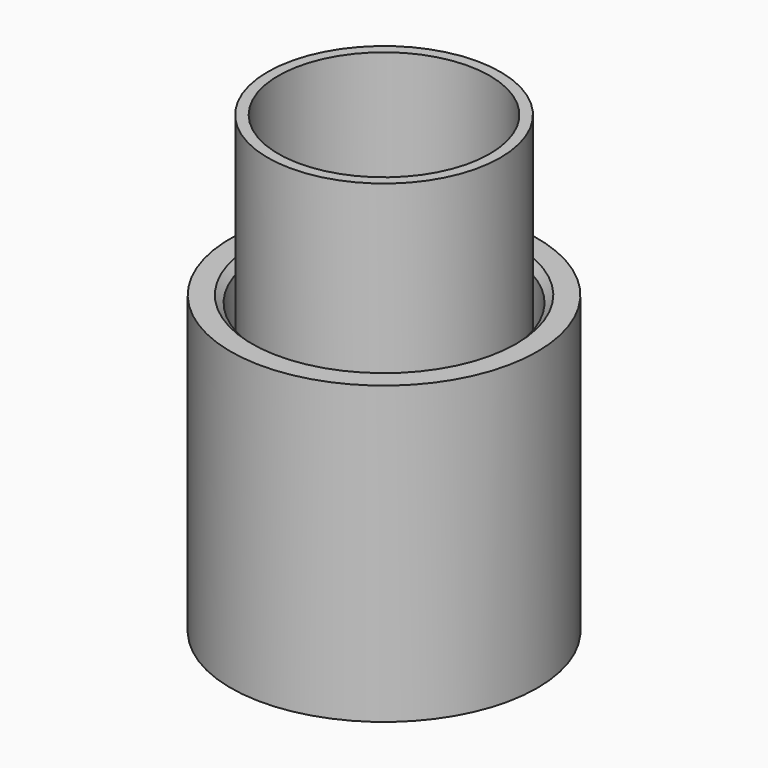
from build123d import *

# Parameters (mm, degrees)
F0_R     = 11
F0_R_2   = 10
F1_DEPTH = 40
F2_R     = 14.5
F2_R_2   = 11.5
F3_DEPTH = 25
F4_R     = 14.5
F5_DEPTH = 3
F6_SIZE  = 1
F7_SIZE2 = 5
F7_SIZE  = 0.5


with BuildPart() as f1:
    # F0 (on Top) → F1 (new body)
    with BuildSketch(Plane.XY):
        Circle(F0_R)
        Circle(F0_R_2, mode=Mode.SUBTRACT)
    extrude(amount=F1_DEPTH)


with BuildPart() as f3:
    # F2 (on Top) → F3 (new body)
    with BuildSketch(Plane.XY):
        Circle(F2_R)
        Circle(F2_R_2, mode=Mode.SUBTRACT)
    extrude(amount=F3_DEPTH)

    # F4 (on Top) → F5 (join)
    with BuildSketch(Plane.XY):
        Circle(F4_R)
    extrude(amount=-F5_DEPTH)

    # F6
    f6_edges = [f3.edges().sort_by_distance(p)[0] for p in [
        (-11.5, 0, 25),
    ]]
    chamfer(f6_edges, length=F6_SIZE)

    # F7
    f7_edges = [f3.edges().sort_by_distance(p)[0] for p in [
        (-11.5, 0, 24),
    ]]
    chamfer(f7_edges, length=F7_SIZE, length2=F7_SIZE2)


solid = Compound([f1.part, f3.part])
